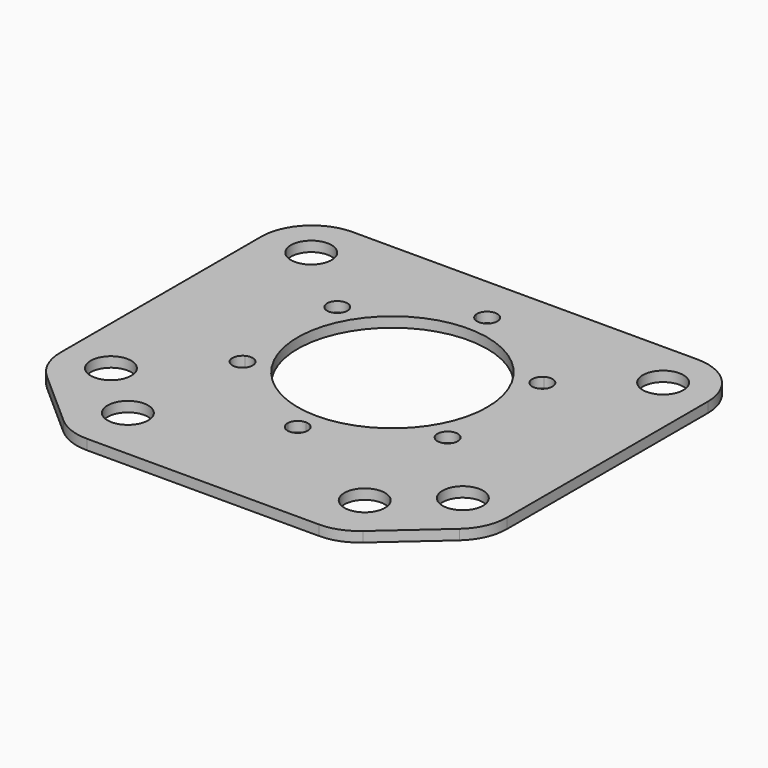
from build123d import *

# Parameters (mm, degrees)
F0_R     = 9
F0_R_2   = 6
F1_DEPTH = 3


# Not quite as in the source:
# - a feature names something its author has since deleted; it is built from what else it names


with BuildPart() as f1:
    # F0 (on Top) → F1 (new body)
    with BuildSketch(Plane.XY):
        with BuildLine():
            ThreePointArc((0, 49), (-49, 0), (0, -49))
            ThreePointArc((0, -49), (34.6482322781, -34.6482322781), (49, 0))
            ThreePointArc((49, 0), (34.6482322781, 34.6482322781), (0, 49))
        make_face()
        with BuildLine():
            ThreePointArc((31.698164825, 14.8400251593), (34.1645706023, 7.601454832), (35, 0))
            ThreePointArc((35, 0), (34.1645706023, -7.601454832), (31.698164825, -14.8400251593))
            ThreePointArc((31.698164825, -14.8400251593), (32.8762182612, -15.9446587316), (33.3108891325, -17.5))
            ThreePointArc((33.3108891325, -17.5), (31.7548586928, -20.1296296144), (28.7009211933, -20.0314034121))
            ThreePointArc((28.7009211933, -20.0314034121), (17.5, -30.3108891325), (2.9972436317, -34.8714285714))
            ThreePointArc((2.9972436317, -34.8714285714), (2.9993108288, -34.9356995144), (3, -35))
            ThreePointArc((3, -35), (2.1213203436, -37.1213203436), (0, -38))
            ThreePointArc((0, -38), (-2.1663003353, -37.0753657165), (-2.9972436317, -34.8714285714))
            ThreePointArc((-2.9972436317, -34.8714285714), (-17.5, -30.3108891325), (-28.7009211933, -20.0314034121))
            ThreePointArc((-28.7009211933, -20.0314034121), (-32.9089653438, -19), (-31.698164825, -14.8400251593))
            ThreePointArc((-31.698164825, -14.8400251593), (-35, 0), (-31.698164825, 14.8400251593))
            ThreePointArc((-31.698164825, 14.8400251593), (-32.9089653438, 19), (-28.7009211933, 20.0314034121))
            ThreePointArc((-28.7009211933, 20.0314034121), (-17.5, 30.3108891325), (-2.9972436317, 34.8714285714))
            ThreePointArc((-2.9972436317, 34.8714285714), (-0.0643004856, 37.9993108288), (3, 35))
            ThreePointArc((3, 35), (2.9993108288, 34.9356995144), (2.9972436317, 34.8714285714))
            ThreePointArc((2.9972436317, 34.8714285714), (17.5, 30.3108891325), (28.7009211933, 20.0314034121))
            ThreePointArc((28.7009211933, 20.0314034121), (31.7548586928, 20.1296296144), (33.3108891325, 17.5))
            ThreePointArc((33.3108891325, 17.5), (32.8762182612, 15.9446587316), (31.698164825, 14.8400251593))
        make_face(mode=Mode.SUBTRACT)
        with BuildLine():
            ThreePointArc((31.698164825, -14.8400251593), (34.1645706023, -7.601454832), (35, 0))
            ThreePointArc((35, 0), (34.1645706023, 7.601454832), (31.698164825, 14.8400251593))
            ThreePointArc((31.698164825, 14.8400251593), (27.7128129211, 16), (28.7009211933, 20.0314034121))
            ThreePointArc((28.7009211933, 20.0314034121), (17.5, 30.3108891325), (2.9972436317, 34.8714285714))
            ThreePointArc((2.9972436317, 34.8714285714), (0, 32), (-2.9972436317, 34.8714285714))
            ThreePointArc((-2.9972436317, 34.8714285714), (-17.5, 30.3108891325), (-28.7009211933, 20.0314034121))
            ThreePointArc((-28.7009211933, 20.0314034121), (-27.6812595181, 18.9439695603), (-27.3108891325, 17.5))
            ThreePointArc((-27.3108891325, 17.5), (-28.755547864, 14.9346708713), (-31.698164825, 14.8400251593))
            ThreePointArc((-31.698164825, 14.8400251593), (-35, 0), (-31.698164825, -14.8400251593))
            ThreePointArc((-31.698164825, -14.8400251593), (-28.755547864, -14.9346708713), (-27.3108891325, -17.5))
            ThreePointArc((-27.3108891325, -17.5), (-27.6812595181, -18.9439695603), (-28.7009211933, -20.0314034121))
            ThreePointArc((-28.7009211933, -20.0314034121), (-17.5, -30.3108891325), (-2.9972436317, -34.8714285714))
            ThreePointArc((-2.9972436317, -34.8714285714), (-2.0753657165, -32.8336996647), (0, -32))
            ThreePointArc((0, -32), (2.0753657165, -32.8336996647), (2.9972436317, -34.8714285714))
            ThreePointArc((2.9972436317, -34.8714285714), (17.5, -30.3108891325), (28.7009211933, -20.0314034121))
            ThreePointArc((28.7009211933, -20.0314034121), (27.7128129211, -16), (31.698164825, -14.8400251593))
        make_face()
        with BuildLine():
            ThreePointArc((28, 0), (19.7989898732, -19.7989898732), (0, -28))
            ThreePointArc((0, -28), (-19.7989898732, 19.7989898732), (28, 0))
        make_face(mode=Mode.SUBTRACT)
        with BuildLine():
            Line((0, -70), (0, -49))
            ThreePointArc((0, -49), (-49, 0), (0, 49))
            Line((0, 49), (-51, 49))
            ThreePointArc((-51, 49), (-61.6066017178, 44.6066017178), (-66, 34))
            Line((-66, 34), (-66, -40.2424365873))
            ThreePointArc((-66, -40.2424365873), (-64.6762407754, -46.4036408731), (-60.938608233, -51.4773850246))
            Line((-60.938608233, -51.4773850246), (-44.2561452447, -66.2349484374))
            ThreePointArc((-44.2561452447, -66.2349484374), (-39.6314702743, -69.0271919243), (-34.3175370117, -70))
            Line((-34.3175370117, -70), (0, -70))
        make_face()
        with Locations((-35, -54)):
            Circle(F0_R, mode=Mode.SUBTRACT)
        with Locations((-52, -39)):
            Circle(F0_R, mode=Mode.SUBTRACT)
        with Locations((-52, 35)):
            Circle(F0_R, mode=Mode.SUBTRACT)
        with BuildLine():
            ThreePointArc((49, 0), (34.6482322781, -34.6482322781), (0, -49))
            Line((0, -49), (0, -70))
            Line((0, -70), (34.3175370117, -70))
            ThreePointArc((34.3175370117, -70), (39.6314702743, -69.0271919243), (44.2561452447, -66.2349484374))
            Line((44.2561452447, -66.2349484374), (60.938608233, -51.4773850246))
            ThreePointArc((60.938608233, -51.4773850246), (64.6762407754, -46.4036408731), (66, -40.2424365873))
            Line((66, -40.2424365873), (66, 34))
            ThreePointArc((66, 34), (61.6066017178, 44.6066017178), (51, 49))
            Line((51, 49), (0, 49))
            ThreePointArc((0, 49), (34.6482322781, 34.6482322781), (49, 0))
        make_face()
        with Locations((35, -54)):
            Circle(F0_R, mode=Mode.SUBTRACT)
        with Locations((52, -39)):
            Circle(F0_R, mode=Mode.SUBTRACT)
        with Locations((52, 35)):
            Circle(F0_R, mode=Mode.SUBTRACT)
        with Locations((-52, 35)):
            Circle(F0_R)
        with Locations((-52, 35)):
            Circle(F0_R_2, mode=Mode.SUBTRACT)
        with Locations((-52, -39)):
            Circle(F0_R)
        with Locations((-52, -39)):
            Circle(F0_R_2, mode=Mode.SUBTRACT)
        with Locations((-35, -54)):
            Circle(F0_R)
        with Locations((-35, -54)):
            Circle(F0_R_2, mode=Mode.SUBTRACT)
        with Locations((35, -54)):
            Circle(F0_R)
        with Locations((35, -54)):
            Circle(F0_R_2, mode=Mode.SUBTRACT)
        with Locations((52, -39)):
            Circle(F0_R)
        with Locations((52, -39)):
            Circle(F0_R_2, mode=Mode.SUBTRACT)
        with Locations((52, 35)):
            Circle(F0_R)
        with Locations((52, 35)):
            Circle(F0_R_2, mode=Mode.SUBTRACT)
    extrude(amount=F1_DEPTH)


solid = f1.part
